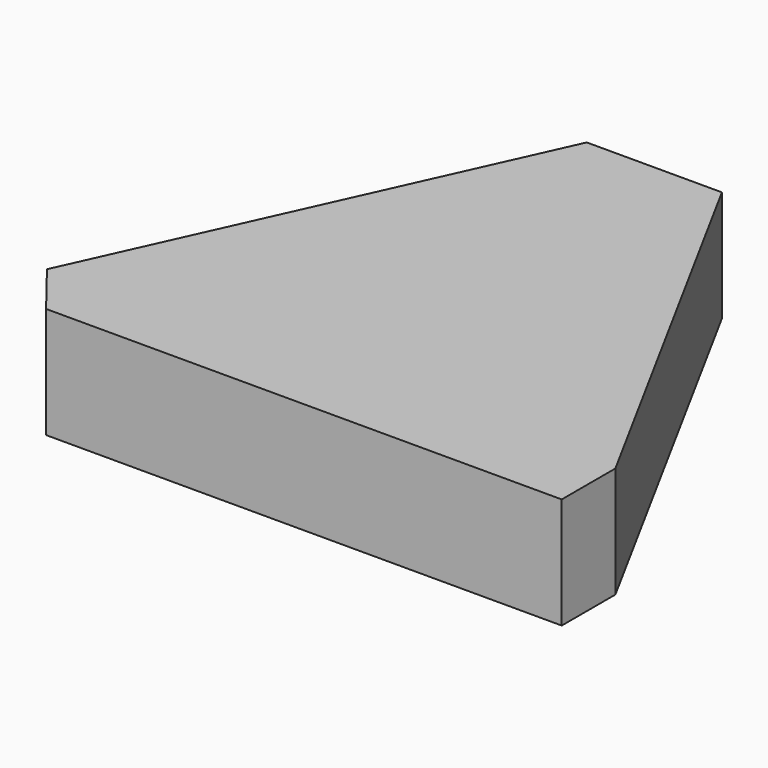
from build123d import *

# Parameters (mm, degrees)
F2_DEPTH    = 21.8264274299
F3_R        = 5.08
F4_T        = -2.54
F5_SIZE     = 12.7
F6_SIZE     = 5.08
F7_SIZE     = 5.08
F8_T1_DEPTH = 70.3417608066


# Not quite as in the source:
# - a fillet or chamfer that OpenCascade refuses, or shapes differently, is made with other operations: its cross-section is extruded or revolved along the edge and cut away or added
# - a shell that OpenCascade refuses in one call is made with other operations: the cavity is built on its own and cut out


with BuildPart() as f2:
    # F1 (on Top) → F2 (new body)
    with BuildSketch(Plane.XY):
        Polygon((-21.634221077, -25.4589989781), (-15.6604591757, -36.3845676184), (26.2466259301, -36.3845676184), (26.2466259301, -26.9864313304), (14.4790392369, -10.1876780391), (-12.1967634186, -10.1876780391), align=None)
    extrude(amount=F2_DEPTH)

    # F5
    f5_edges = [f2.edges().sort_by_distance(p)[0] for p in [
        (1.141138, -10.187678, 0),
    ]]
    chamfer(f5_edges, length=F5_SIZE)

    # F6
    f6_edges = [f2.edges().sort_by_distance(p)[0] for p in [
        (1.665127, -22.887678, 0),
    ]]
    chamfer(f6_edges, length=F6_SIZE)

    # F7
    f7_edges = [f2.edges().sort_by_distance(p)[0] for p in [
        (2.992036, -27.967678, 0),
    ]]
    chamfer(f7_edges, length=F7_SIZE)

    # F8: chamfer of 5.08 on 1 edges, made by hand

    # F8_s2 → F8_t1 (cut)
    with BuildSketch(Plane.YZ.offset(-33.4897993752)):
        Polygon((-18.5810619888, 3.8880636728), (-28.2567592384, 0.9529730006), (-23.2743700139, 1.9440318364), align=None)
    extrude(amount=F8_T1_DEPTH, mode=Mode.SUBTRACT)


with BuildPart() as f2b:
    # F0 (on Top) → F2, piece 2 (new body)
    with BuildSketch(Plane.XY):
        Polygon((15.5484518036, 53.0691556633), (-11.0087171197, 53.0691556633), (-49.3722259998, -31.5896049142), (-41.2309654057, -41.9769249856), (60.1042881608, -41.9769249856), (60.1042881608, -28.8013797253), align=None)
    extrude(amount=F2_DEPTH)

    # F3
    f3_edges = [f2b.edges().sort_by_distance(p)[0] for p in [
        (-30.190472, 10.739775, 0),
    ]]
    fillet(f3_edges, radius=F3_R)

    # F4: a shell. OpenCascade refuses it in one call, so the cavity is built on its own and cut out:
    # the body offset inwards by the wall thickness, plus a prism from it out through each open face.
    f4_core = offset(f2b.part, amount=F4_T, kind=Kind.INTERSECTION, mode=Mode.PRIVATE)
    f4_exits = [f4_core.faces().sort_by_distance(p)[0] for p in [
        (6.185491, -4.45819, 2.54),
    ]]
    add(f4_core, mode=Mode.SUBTRACT)
    extrude(f4_exits, amount=-F4_T, mode=Mode.SUBTRACT)


solid = Compound([f2.part, f2b.part])
